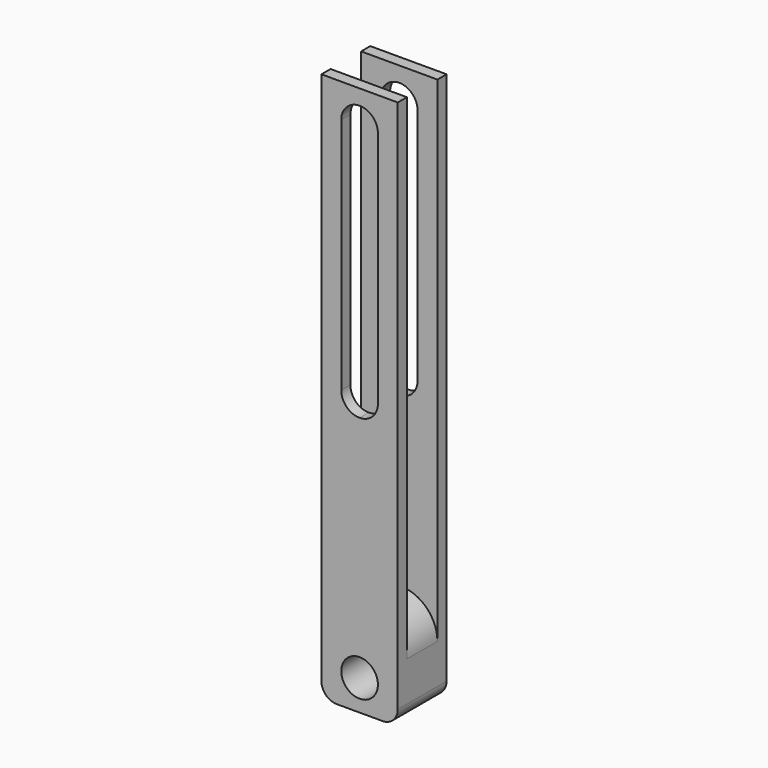
from build123d import *

# Parameters (mm, degrees)
F1_DEPTH = 12.5
F2_R     = 6
F3_DEPTH = 20.001
F4_R     = 5
F5_R     = 12
F6_W     = 12
F6_H     = 90
F7_DEPTH = 20.001
F8_R     = 5.99999


# Not quite as in the source:
# - a fillet or chamfer is up to 0.001 mm smaller than in the source, because OpenCascade refuses the exact size


with BuildPart() as f1:
    # F0 (on Right) → F1 (new body, symmetric)
    with BuildSketch(Plane.YZ):
        Polygon((-6.25, 170), (-10, 170), (-10, -10), (10, -10), (10, 170), (6.25, 170), (6.25, 20), (-6.25, 20), align=None)
    extrude(amount=F1_DEPTH, both=True)

    # F2 (on face) → F3 (cut, through all)
    with BuildSketch(Plane.XZ.offset(10)):
        Circle(F2_R)
    extrude(amount=-F3_DEPTH, mode=Mode.SUBTRACT)

    # F4
    f4_edges = [f1.edges().sort_by_distance(p)[0] for p in [
        (12.5, 0, -10),
        (-12.5, 0, -10),
    ]]
    fillet(f4_edges, radius=F4_R)

    # F5
    f5_edges = [f1.edges().sort_by_distance(p)[0] for p in [
        (12.5, 0, 20),
        (-12.5, 0, 20),
    ]]
    fillet(f5_edges, radius=F5_R)

    # F6 (on face) → F7 (cut, through all)
    with BuildSketch(Plane.XZ.offset(10)):
        with Locations((0, 120)):
            Rectangle(F6_W, F6_H)
    extrude(amount=-F7_DEPTH, mode=Mode.SUBTRACT)

    # F8 (radius 6 in the source; OpenCascade refuses exactly that, so slightly less here)
    f8_edges = [f1.edges().sort_by_distance(p)[0] for p in [
        (-6, -8.125, 165),
        (6, -8.125, 165),
        (6, -8.125, 75),
        (-6, -8.125, 75),
        (-6, 8.125, 75),
        (6, 8.125, 75),
        (6, 8.125, 165),
        (-6, 8.125, 165),
    ]]
    fillet(f8_edges, radius=F8_R)


solid = f1.part
